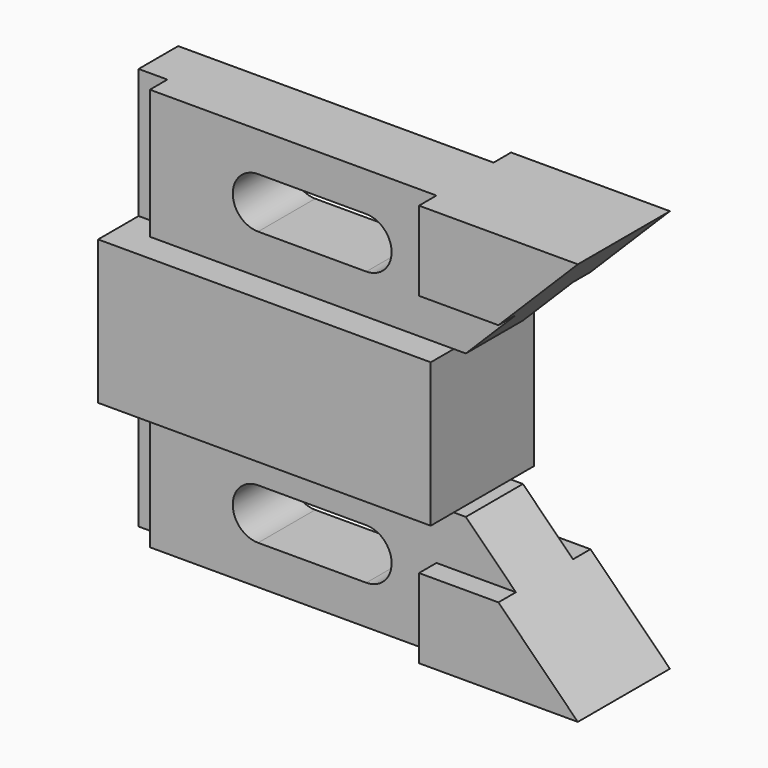
from build123d import *

# Parameters (mm, degrees)
F0_W     = 28.448
F0_H     = 31.75
F1_DEPTH = 73.406
F3_DEPTH = 7.874
F4_W     = 6.35
F4_H     = 28.575
F5_DEPTH = 4.826
F7_DEPTH = 12.7


# Not quite as in the source:
# - a pattern or mirror of a feature is missing from the dataset's text; its kind, count and spacing are read off the source's solid


with BuildPart() as f1:
    # F0 (on Right) → F1 (new body)
    with BuildSketch(Plane.YZ):
        Rectangle(F0_W, F0_H)
    extrude(amount=F1_DEPTH)

    # F2 (on Front) → F3 (join, symmetric)
    with BuildSketch(Plane.XZ):
        Polygon((0, 15.875), (76.073, 15.875), (104.648, 44.45), (0, 44.45), align=None)
        with BuildLine():
            ThreePointArc((30.226, 24.638), (24.638, 30.226), (30.226, 35.814))
            Line((30.226, 35.814), (54.102, 35.814))
            ThreePointArc((54.102, 35.814), (58.0533126933, 34.1773126933), (59.69, 30.226))
            ThreePointArc((59.69, 30.226), (58.0533126933, 26.2746873067), (54.102, 24.638))
            Line((54.102, 24.638), (30.226, 24.638))
        make_face(mode=Mode.SUBTRACT)
        Polygon((76.073, -15.875), (0, -15.875), (0, -44.45), (104.648, -44.45), align=None)
        with BuildLine():
            ThreePointArc((54.102, -24.638), (58.0533126933, -26.2746873067), (59.69, -30.226))
            ThreePointArc((59.69, -30.226), (58.0533126933, -34.1773126933), (54.102, -35.814))
            Line((54.102, -35.814), (30.226, -35.814))
            ThreePointArc((30.226, -35.814), (24.638, -30.226), (30.226, -24.638))
            Line((30.226, -24.638), (54.102, -24.638))
        make_face(mode=Mode.SUBTRACT)
    extrude(amount=F3_DEPTH, both=True)

    # F4 (on face) → F5 (cut)
    with BuildSketch(Plane.XZ.offset(7.874)):
        with Locations((3.175, 30.1625)):
            Rectangle(F4_W, F4_H)
    f5 = extrude(amount=-F5_DEPTH, mode=Mode.SUBTRACT)

    # F5_copies: F5 across plane
    add(f5.mirror(Plane(origin=(0, 0, 0), x_dir=(-1, 0, 0), z_dir=(0, 0, -1))), mode=Mode.SUBTRACT)

    # F6 (on Front) → F7 (join, symmetric)
    with BuildSketch(Plane.XZ):
        Polygon((104.648, 44.45), (69.596, 44.45), (69.596, 26.924), (87.122, 26.924), align=None)
    f7 = extrude(amount=F7_DEPTH, both=True)

    # F7_copies: F7 across plane
    add(f7.mirror(Plane(origin=(0, 0, 0), x_dir=(-1, 0, 0), z_dir=(0, 0, -1))))


solid = f1.part
